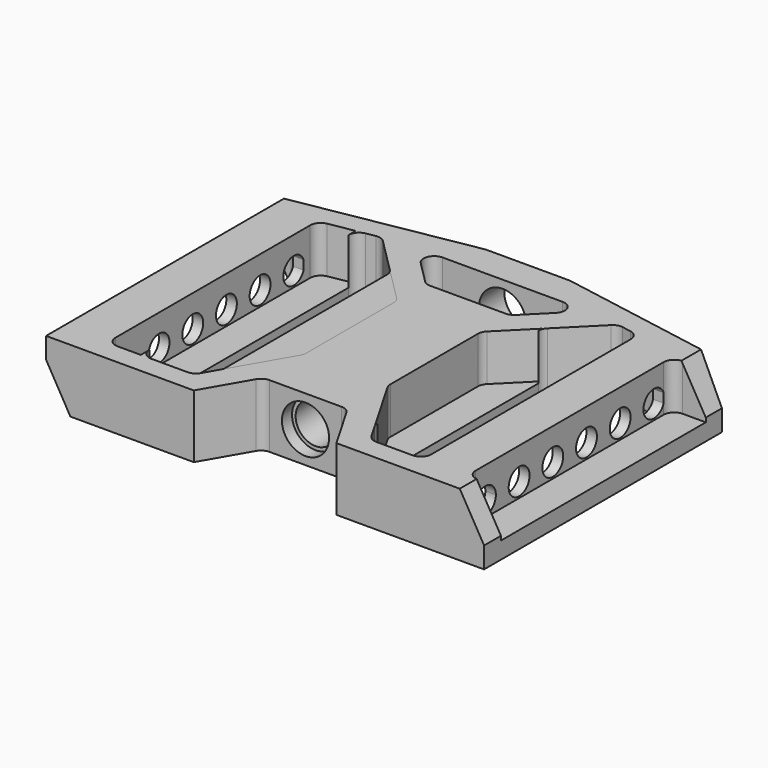
from build123d import *

# Parameters (mm, degrees)
F6_DEPTH       = 9.525
F7_DEPTH       = 19.051
F8_DEPTH       = 19.051
F9_DEPTH       = 13.97
F10_DEPTH      = 13.97
F11_DEPTH      = 13.97
F18_DEPTH      = 9.525
F19_DEPTH      = 9.525
F20_DEPTH      = 9.525
F21_DEPTH      = 9.525
F21_DEPTH_BACK = 4.445
F22_DEPTH      = 9.525
F22_DEPTH_BACK = 4.445
F23_DEPTH      = 9.525
F23_DEPTH_BACK = 4.445
F24_R          = 3.937
F25_DEPTH      = 3.175
F26_R          = 3.937
F27_DEPTH      = 3.175
F28_R          = 4.318
F29_DEPTH      = 83.821
F30_R          = 6.0325
F31_DEPTH      = 13.97
F32_R          = 7.112
F33_DEPTH      = 3.81
F34_R          = 6.4897
F34_R_2        = 4.318
F35_DEPTH      = 35.56
F36_R          = 6.731
F37_DEPTH      = 31.369
F38_R          = 7.112
F39_DEPTH      = 24.384
F41_DEPTH      = 99.061
F43_DEPTH      = 99.061


with BuildPart() as f6:
    # F1 (on Top) → F6 (new body, symmetric)
    with BuildSketch(Plane.XY):
        with BuildLine():
            Line((0, 89.654718849), (0, 0))
            Line((0, 0), (44.5411818976, 0))
            Line((44.5411818976, 0), (52.4234564477, 13.6525))
            ThreePointArc((52.4234564477, 13.6525), (53.5855871047, 14.814630657), (55.1730871047, 15.24))
            Line((55.1730871047, 15.24), (66.04, 15.24))
            Line((66.04, 15.24), (66.04, 99.06))
            Line((66.04, 99.06), (53.34, 99.06))
            Line((53.34, 99.06), (0, 89.654718849))
        make_face()
    extrude(amount=F6_DEPTH, both=True)


with BuildPart() as f6b:
    # F2 (on face) → F6, piece 2 (new body, symmetric)
    with BuildSketch(Plane.XY):
        with BuildLine():
            Line((52.4100640303, 66.6076286244), (43.18, 75.8376926547))
            Line((43.18, 75.8376926547), (43.18, 12.8823637951))
            Line((43.18, 12.8823637951), (52.914630657, 29.743238686))
            ThreePointArc((52.914630657, 29.743238686), (53.2318144985, 30.5089882178), (53.34, 31.330738686))
            Line((53.34, 31.330738686), (53.34, 64.3625645942))
            ThreePointArc((53.34, 64.3625645942), (53.0983175157, 65.5775844919), (52.4100640303, 66.6076286244))
        make_face()
    extrude(amount=F6_DEPTH, both=True)


with BuildPart() as f6c:
    # F4 (on face) → F6, piece 3 (new body, symmetric)
    with BuildSketch(Plane.XY):
        with BuildLine():
            Line((23.495, 6.35), (23.495, 87.3495622753))
            Line((23.495, 87.3495622753), (15.9586670359, 86.0207034381))
            ThreePointArc((15.9586670359, 86.0207034381), (14.0778088931, 84.9347894831), (13.335, 82.8939388223))
            Line((13.335, 82.8939388223), (13.335, 9.525))
            ThreePointArc((13.335, 9.525), (14.2649359697, 7.2799359697), (16.51, 6.35))
            Line((16.51, 6.35), (23.495, 6.35))
        make_face()
    extrude(amount=F6_DEPTH, both=True)


with BuildPart() as f6d:
    # F5 (on face) → F6, piece 4 (new body, symmetric)
    with BuildSketch(Plane.XY):
        with BuildLine():
            Line((6.985, 83.566), (0, 83.566))
            Line((0, 83.566), (0, 6.35))
            Line((0, 6.35), (6.985, 6.35))
            ThreePointArc((6.985, 6.35), (9.2300640303, 7.2799359697), (10.16, 9.525))
            Line((10.16, 9.525), (10.16, 80.391))
            ThreePointArc((10.16, 80.391), (9.2300640303, 82.6360640303), (6.985, 83.566))
        make_face()
    extrude(amount=F6_DEPTH, both=True)


with BuildPart() as f6e:
    # F0 (on Top) → F6, piece 5 (new body, symmetric)
    with BuildSketch(Plane.XY):
        with BuildLine():
            Line((66.04, 76.454), (66.04, 89.535))
            Line((66.04, 89.535), (47.9241280605, 89.535))
            ThreePointArc((47.9241280605, 89.535), (44.9908105448, 87.5750198978), (45.6790640303, 84.1149359697))
            Line((45.6790640303, 84.1149359697), (52.4100640303, 77.3839359697))
            ThreePointArc((52.4100640303, 77.3839359697), (53.4401081628, 76.6956824843), (54.6551280605, 76.454))
            Line((54.6551280605, 76.454), (66.04, 76.454))
        make_face()
    extrude(amount=F6_DEPTH, both=True)


with BuildPart() as f6f:
    # F3 (on face) → F6, piece 6 (new body, symmetric)
    with BuildSketch(Plane.XY):
        with BuildLine():
            ThreePointArc((43.18, 74.5225645942), (42.9383175157, 75.7375844919), (42.2500640303, 76.7676286244))
            Line((42.2500640303, 76.7676286244), (31.6117153015, 87.4059773532))
            ThreePointArc((31.6117153015, 87.4059773532), (30.3213921846, 88.1889646416), (28.8153183071, 88.2876779388))
            Line((28.8153183071, 88.2876779388), (26.1186670359, 87.8121855621))
            ThreePointArc((26.1186670359, 87.8121855621), (24.2378088931, 86.726271607), (23.495, 84.6854209463))
            Line((23.495, 84.6854209463), (23.495, 9.525))
            ThreePointArc((23.495, 9.525), (24.4249359697, 7.2799359697), (26.67, 6.35))
            Line((26.67, 6.35), (37.5754508998, 6.35))
            ThreePointArc((37.5754508998, 6.35), (39.1629508998, 6.775369343), (40.3250815568, 7.9375))
            Line((40.3250815568, 7.9375), (42.7546306556, 12.1456024786))
            ThreePointArc((42.7546306556, 12.1456024786), (36.9381855019, 14.5548529507), (43.18, 13.7331024811))
            Line((43.18, 13.7331024811), (43.18, 74.5225645942))
        make_face()
        with BuildLine():
            ThreePointArc((42.7546306556, 12.1456024786), (43.0718144981, 12.9113520115), (43.18, 13.7331024811))
            ThreePointArc((43.18, 13.7331024811), (36.9381855019, 14.5548529507), (42.7546306556, 12.1456024786))
        make_face()
        with BuildLine():
            Line((43.18, 12.8823637951), (43.18, 13.7331024811))
            ThreePointArc((43.18, 13.7331024811), (43.0718144981, 12.9113520115), (42.7546306556, 12.1456024786))
            Line((42.7546306556, 12.1456024786), (43.18, 12.8823637951))
        make_face()
    extrude(amount=F6_DEPTH, both=True)


with BuildPart() as f7_tool:
    # F7 (cut, through all): a face of the model
    f7_faces = [f6e.part.faces().sort_by_distance(p)[0] for p in [
        (56.697252015, 83.5132399771, 9.525),
    ]]
    extrude(f7_faces, amount=-F7_DEPTH)


with BuildPart() as f6_1:
    add(f6.part)

    # F7: cut by f7_tool
    add(f7_tool.part, mode=Mode.SUBTRACT)


with BuildPart() as f6e_1:
    add(f6e.part)

    # F7: cut by f7_tool
    add(f7_tool.part, mode=Mode.SUBTRACT)


with BuildPart() as f8_tool:
    # F8 (cut, through all): a face of the model
    f8_faces = [f6f.part.faces().sort_by_distance(p)[0] for p in [
        (33.0084850177, 45.7122360619, 9.525),
    ]]
    extrude(f8_faces, amount=-F8_DEPTH)


with BuildPart() as f6_2:
    add(f6_1.part)

    # F8: cut by f8_tool
    add(f8_tool.part, mode=Mode.SUBTRACT)


with BuildPart() as f6f_1:
    add(f6f.part)

    # F8: cut by f8_tool
    add(f8_tool.part, mode=Mode.SUBTRACT)


with BuildPart() as f9_tool:
    # F9 (cut): a face of the model
    f9_faces = [f6c.part.faces().sort_by_distance(p)[0] for p in [
        (18.4535943908, 46.4407977567, 9.525),
    ]]
    extrude(f9_faces, amount=-F9_DEPTH)


with BuildPart() as f6_3:
    add(f6_2.part)

    # F9: cut by f9_tool
    add(f9_tool.part, mode=Mode.SUBTRACT)


with BuildPart() as f6c_1:
    add(f6c.part)

    # F9: cut by f9_tool
    add(f9_tool.part, mode=Mode.SUBTRACT)


with BuildPart() as f10_tool:
    # F10 (cut): a face of the model
    f10_faces = [f6d.part.faces().sort_by_distance(p)[0] for p in [
        (5.0557610793, 44.958, -9.525),
    ]]
    extrude(f10_faces, amount=-F10_DEPTH)


with BuildPart() as f6_4:
    add(f6_3.part)

    # F10: cut by f10_tool
    add(f10_tool.part, mode=Mode.SUBTRACT)


with BuildPart() as f6d_1:
    add(f6d.part)

    # F10: cut by f10_tool
    add(f10_tool.part, mode=Mode.SUBTRACT)


with BuildPart() as f11_tool:
    # F11 (cut): a face of the model
    f11_faces = [f6b.part.faces().sort_by_distance(p)[0] for p in [
        (47.7781090574, 46.0375803763, -9.525),
    ]]
    extrude(f11_faces, amount=-F11_DEPTH)


with BuildPart() as f6_5:
    add(f6_4.part)

    # F11: cut by f11_tool
    add(f11_tool.part, mode=Mode.SUBTRACT)

    # F12 (on Top) → F18 (join, symmetric)
    with BuildSketch(Plane.XY):
        with BuildLine():
            Line((66.04, 99.06), (66.04, 15.24))
            Line((66.04, 15.24), (76.9069128953, 15.24))
            ThreePointArc((76.9069128953, 15.24), (78.4944128953, 14.814630657), (79.6565435523, 13.6525))
            Line((79.6565435523, 13.6525), (87.5388181024, 0))
            Line((87.5388181024, 0), (132.08, 0))
            Line((132.08, 0), (132.08, 89.654718849))
            Line((132.08, 89.654718849), (78.74, 99.06))
            Line((78.74, 99.06), (66.04, 99.06))
        make_face()
    extrude(amount=F18_DEPTH, both=True)

    # F13 (on face) → F19 (cut, symmetric)
    with BuildSketch(Plane.XY):
        with BuildLine():
            Line((84.1558719395, 89.535), (66.04, 89.535))
            Line((66.04, 89.535), (66.04, 76.454))
            Line((66.04, 76.454), (77.4248719395, 76.454))
            ThreePointArc((77.4248719395, 76.454), (78.6398918372, 76.6956824843), (79.6699359697, 77.3839359697))
            Line((79.6699359697, 77.3839359697), (86.4009359697, 84.1149359697))
            ThreePointArc((86.4009359697, 84.1149359697), (87.0891894552, 87.5750198978), (84.1558719395, 89.535))
        make_face()
    extrude(amount=F19_DEPTH, both=True, mode=Mode.SUBTRACT)

    # F15 (on face) → F20 (cut, symmetric)
    with BuildSketch(Plane.XY):
        with BuildLine():
            Line((100.4682846985, 87.4059773532), (89.8299359697, 76.7676286244))
            ThreePointArc((89.8299359697, 76.7676286244), (89.1416824843, 75.7375844919), (88.9, 74.5225645942))
            Line((88.9, 74.5225645942), (88.9, 13.7331024811))
            ThreePointArc((88.9, 13.7331024811), (89.0081855015, 12.9113520129), (89.325369343, 12.1456024811))
            Line((89.325369343, 12.1456024811), (91.7549184432, 7.9375))
            ThreePointArc((91.7549184432, 7.9375), (92.9170491002, 6.775369343), (94.5045491002, 6.35))
            Line((94.5045491002, 6.35), (105.41, 6.35))
            ThreePointArc((105.41, 6.35), (107.6550640303, 7.2799359697), (108.585, 9.525))
            Line((108.585, 9.525), (108.585, 84.6854209463))
            ThreePointArc((108.585, 84.6854209463), (107.8421911069, 86.726271607), (105.9613329641, 87.8121855621))
            Line((105.9613329641, 87.8121855621), (103.2646816929, 88.2876779388))
            ThreePointArc((103.2646816929, 88.2876779388), (101.7586078154, 88.1889646416), (100.4682846985, 87.4059773532))
        make_face()
    extrude(amount=F20_DEPTH, both=True, mode=Mode.SUBTRACT)

    # F14 (on face) → F21 (cut, two sides)
    with BuildSketch(Plane.XY) as f21_sk:
        with BuildLine():
            Line((88.9, 12.8823637951), (88.9, 75.8376926547))
            Line((88.9, 75.8376926547), (79.6699359697, 66.6076286244))
            ThreePointArc((79.6699359697, 66.6076286244), (78.9816824843, 65.5775844919), (78.74, 64.3625645942))
            Line((78.74, 64.3625645942), (78.74, 31.330738686))
            ThreePointArc((78.74, 31.330738686), (78.8481855015, 30.5089882178), (79.165369343, 29.743238686))
            Line((79.165369343, 29.743238686), (88.9, 12.8823637951))
        make_face()
    extrude(amount=F21_DEPTH, mode=Mode.SUBTRACT)
    extrude(f21_sk.sketch, amount=-F21_DEPTH_BACK, mode=Mode.SUBTRACT)

    # F16 (on face) → F22 (cut, two sides)
    with BuildSketch(Plane.XY) as f22_sk:
        with BuildLine():
            Line((116.1213329641, 86.0207034381), (108.585, 87.3495622753))
            Line((108.585, 87.3495622753), (108.585, 6.35))
            Line((108.585, 6.35), (115.57, 6.35))
            ThreePointArc((115.57, 6.35), (117.8150640303, 7.2799359697), (118.745, 9.525))
            Line((118.745, 9.525), (118.745, 82.8939388223))
            ThreePointArc((118.745, 82.8939388223), (118.0021911069, 84.9347894831), (116.1213329641, 86.0207034381))
        make_face()
    extrude(amount=-F22_DEPTH, mode=Mode.SUBTRACT)
    extrude(f22_sk.sketch, amount=F22_DEPTH_BACK, mode=Mode.SUBTRACT)

    # F17 (on face) → F23 (cut, two sides)
    with BuildSketch(Plane.XY) as f23_sk:
        with BuildLine():
            Line((132.08, 6.35), (132.08, 83.566))
            Line((132.08, 83.566), (125.095, 83.566))
            ThreePointArc((125.095, 83.566), (122.8499359697, 82.6360640303), (121.92, 80.391))
            Line((121.92, 80.391), (121.92, 9.525))
            ThreePointArc((121.92, 9.525), (122.8499359697, 7.2799359697), (125.095, 6.35))
            Line((125.095, 6.35), (132.08, 6.35))
        make_face()
    extrude(amount=F23_DEPTH, mode=Mode.SUBTRACT)
    extrude(f23_sk.sketch, amount=-F23_DEPTH_BACK, mode=Mode.SUBTRACT)

    # F24 (on face) → F25 (cut)
    with BuildSketch(Plane(origin=(10.16, 0, 0), x_dir=(0, -1, 0), z_dir=(-1, 0, 0))):
        with BuildLine():
            Line((-9.525, -1.3912152961), (-9.525, 1.3912152961))
            ThreePointArc((-9.525, 1.3912152961), (-17.145, 0), (-9.525, -1.3912152961))
        make_face()
        with BuildLine():
            ThreePointArc((-72.771, 0), (-76.0008939259, 3.8729794732), (-80.391, 1.3912152961))
            Line((-80.391, 1.3912152961), (-80.391, -1.3912152961))
            ThreePointArc((-80.391, -1.3912152961), (-76.0008939259, -3.8729794732), (-72.771, 0))
        make_face()
        with Locations((-25.908, 0)):
            Circle(F24_R)
        with Locations((-38.608, 0)):
            Circle(F24_R)
        with Locations((-51.308, 0)):
            Circle(F24_R)
        with Locations((-64.008, 0)):
            Circle(F24_R)
    extrude(amount=-F25_DEPTH, mode=Mode.SUBTRACT)

    # F26 (on face) → F27 (cut)
    with BuildSketch(Plane.YZ.offset(121.92)):
        with BuildLine():
            ThreePointArc((9.525, -1.3912152961), (13.9151060741, -3.8729794732), (17.145, 0))
            ThreePointArc((17.145, 0), (13.9151060741, 3.8729794732), (9.525, 1.3912152961))
            Line((9.525, 1.3912152961), (9.525, -1.3912152961))
        make_face()
        with BuildLine():
            Line((80.391, -1.3912152961), (80.391, 1.3912152961))
            ThreePointArc((80.391, 1.3912152961), (72.771, 0), (80.391, -1.3912152961))
        make_face()
        with Locations((25.908, 0)):
            Circle(F26_R)
        with Locations((38.608, 0)):
            Circle(F26_R)
        with Locations((51.308, 0)):
            Circle(F26_R)
        with Locations((64.008, 0)):
            Circle(F26_R)
    extrude(amount=-F27_DEPTH, mode=Mode.SUBTRACT)

    # F28 (on face) → F29 (cut, through all)
    with BuildSketch(Plane.XZ.offset(-15.24)):
        with Locations((66.04, 0)):
            Circle(F28_R)
    extrude(amount=-F29_DEPTH, mode=Mode.SUBTRACT)

    # F30 (on face) → F31 (cut)
    with BuildSketch(Plane.XZ.offset(-15.24)):
        with Locations((66.04, 0)):
            Circle(F30_R)
    extrude(amount=-F31_DEPTH, mode=Mode.SUBTRACT)

    # F32 (on face) → F33 (cut)
    with BuildSketch(Plane.XZ.offset(-15.24)):
        with Locations((66.04, 0)):
            Circle(F32_R)
    extrude(amount=-F33_DEPTH, mode=Mode.SUBTRACT)

    # F34 (on face) → F35 (cut)
    with BuildSketch(Plane(origin=(0, 99.06, 0), x_dir=(-1, 0, 0), z_dir=(0, 1, 0))):
        with Locations((-66.04, 0)):
            Circle(F34_R)
        with Locations((-66.04, 0)):
            Circle(F34_R_2, mode=Mode.SUBTRACT)
    extrude(amount=-F35_DEPTH, mode=Mode.SUBTRACT)

    # F36 (on face) → F37 (cut)
    with BuildSketch(Plane(origin=(0, 99.06, 0), x_dir=(-1, 0, 0), z_dir=(0, 1, 0))):
        with Locations((-66.04, 0)):
            Circle(F36_R)
    extrude(amount=-F37_DEPTH, mode=Mode.SUBTRACT)

    # F38 (on face) → F39 (cut)
    with BuildSketch(Plane(origin=(0, 99.06, 0), x_dir=(-1, 0, 0), z_dir=(0, 1, 0))):
        with Locations((-66.04, 0)):
            Circle(F38_R)
    extrude(amount=-F39_DEPTH, mode=Mode.SUBTRACT)

    # F40 (on face) → F41 (cut, through all)
    with BuildSketch(Plane.XZ):
        Polygon((7.3323484187, -9.525), (0, 3.175), (0, -9.525), align=None)
    extrude(amount=-F41_DEPTH, mode=Mode.SUBTRACT)

    # F42 (on face) → F43 (cut, through all)
    with BuildSketch(Plane.XZ):
        Polygon((124.7476515813, 9.525), (132.08, -3.175), (132.08, 9.525), align=None)
    extrude(amount=-F43_DEPTH, mode=Mode.SUBTRACT)


with BuildPart() as f6b_1:
    add(f6b.part)

    # F11: cut by f11_tool
    add(f11_tool.part, mode=Mode.SUBTRACT)


solid = Compound([f6c_1.part, f6d_1.part, f6_5.part, f6b_1.part])
